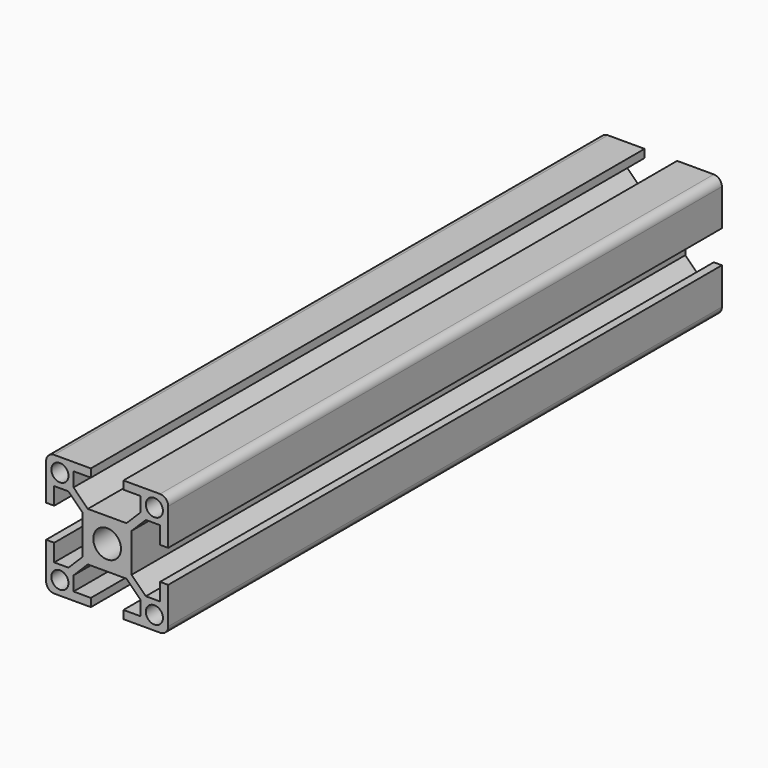
from build123d import *

# Parameters (mm, degrees)
F1_DEPTH = 170
F2_DEPTH = 400
F3_W     = 18.6485039899
F3_H     = 8
F3_W_2   = 19.9612321942
F3_R     = 3.4
F3_R_2   = 2.1
F4_DEPTH = 170
F5_R     = 2


# Not quite as in the source:
# - a pattern or mirror of a feature is missing from the dataset's text; its kind, count and spacing are read off the source's solid


with BuildPart() as f1:
    # F0 (on Front) → F1 (new body)
    with BuildSketch(Plane.XZ):
        Polygon((15, -15), (15, 15), (4, 15), (4, 13), (8.25, 13), (8.25, 9.5), (4.75, 6), (-4.75, 6), (-8.25, 9.5), (-8.25, 13), (-4, 13), (-4, 15), (-15, 15), (-15, -15), align=None)
        Polygon((4, 13), (4, 15), (-4, 15), (-4, 13), (-8.25, 13), (-8.25, 9.5), (-4.75, 6), (4.75, 6), (8.25, 9.5), (8.25, 13), align=None)
    extrude(amount=F1_DEPTH)

    # F0 (on Front) → F2 (cut)
    with BuildSketch(Plane.XZ):
        Polygon((4, 13), (4, 15), (-4, 15), (-4, 13), (-8.25, 13), (-8.25, 9.5), (-4.75, 6), (4.75, 6), (8.25, 9.5), (8.25, 13), align=None)
    f2 = extrude(amount=F2_DEPTH, mode=Mode.SUBTRACT)

    # F2_copies: F2 across plane
    add(f2.mirror(Plane(origin=(0, 0, 0), x_dir=(-1, 0, 0), z_dir=(0, 0, -1))), mode=Mode.SUBTRACT)

    # F3 (on face) → F4 (cut)
    with BuildSketch(Plane(origin=(0, 0, 0), x_dir=(-1, 0, 0), z_dir=(0, 1, 0))):
        Polygon((-6, 4.75), (-9.5, 8.25), (-13, 8.25), (-13, 4), (-13, -4), (-13, -8.25), (-9.5, -8.25), (-6, -4.75), align=None)
        with Locations((-22.3242519949, 0)):
            Rectangle(F3_W, F3_H)
        Polygon((13, 8.25), (9.5, 8.25), (6, 4.75), (6, -4.75), (9.5, -8.25), (13, -8.25), (13, -4), (13, 4), align=None)
        with Locations((22.9806160971, 0)):
            Rectangle(F3_W_2, F3_H)
        Circle(F3_R)
        with Locations((-11.6, 11.6)):
            Circle(F3_R_2)
        with Locations((-11.6, -11.6)):
            Circle(F3_R_2)
        with Locations((11.6, -11.6)):
            Circle(F3_R_2)
        with Locations((11.6, 11.6)):
            Circle(F3_R_2)
    extrude(amount=-F4_DEPTH, mode=Mode.SUBTRACT)

    # F5
    f5_edges = [f1.edges().sort_by_distance(p)[0] for p in [
        (-15, -85, 15),
        (-15, -85, -15),
        (15, -85, -15),
        (15, -85, 15),
    ]]
    fillet(f5_edges, radius=F5_R)


solid = f1.part
